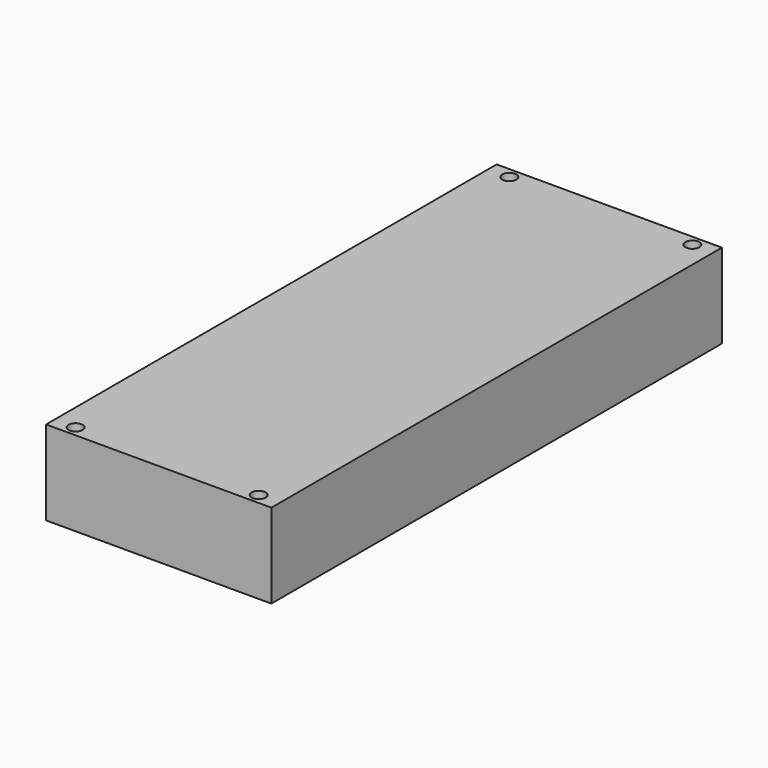
from build123d import *

# Parameters (mm, degrees)
F0_W     = 25.4
F0_H     = 63.5
F0_R     = 0.79375
F1_DEPTH = 4.7625


# Not quite as in the source:
# - a length typed as a fraction of an inch, garbled in the dataset ("3 / 203.2 mm" for 3/8 in), is restored


with BuildPart() as f1:
    # F0 (on Top) → F1 (new body, symmetric)
    with BuildSketch(Plane.XY):
        Rectangle(F0_W, F0_H)
        with Locations((-10.31875, -30.559375)):
            Circle(F0_R, mode=Mode.SUBTRACT)
        with Locations((10.31875, -30.559375)):
            Circle(F0_R, mode=Mode.SUBTRACT)
        with Locations((-10.31875, 30.559375)):
            Circle(F0_R, mode=Mode.SUBTRACT)
        with Locations((10.31875, 30.559375)):
            Circle(F0_R, mode=Mode.SUBTRACT)
    extrude(amount=F1_DEPTH, both=True)


solid = f1.part
